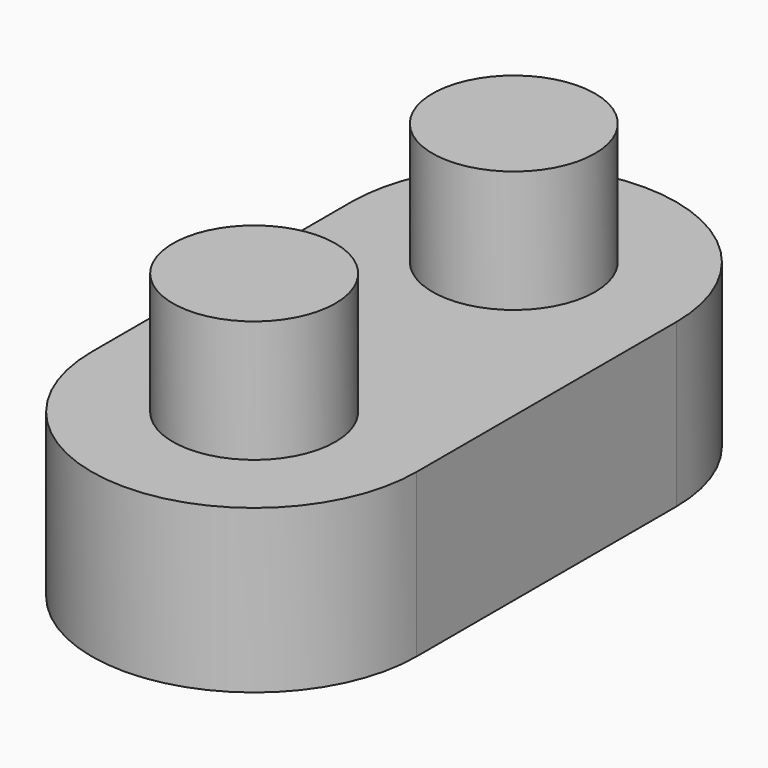
from build123d import *

# Parameters (mm, degrees)
F0_R     = 1
F1_DEPTH = 3.5
F2_DEPTH = 2
F3_DEPTH = 2


# Not quite as in the source:
# - a feature names something its author has since deleted; it is built from what else it names


with BuildPart() as f1:
    # F0 (on Top) → F1 (new body)
    with BuildSketch(Plane.XY):
        with Locations((-2.3999998812, 1.8953582125)):
            Circle(F0_R)
    extrude(amount=F1_DEPTH)



with BuildPart() as f1b:
    # F0 (on Top) → F1, piece 2 (new body)
    with BuildSketch(Plane.XY):
        with Locations((-2.3991598333, -2.1004185153)):
            Circle(F0_R)
    extrude(amount=F1_DEPTH)


with BuildPart() as f1_1:
    add(f1.part)

    add(f1b.part)  # F2 merges F1b
    # F0 (on Top) → F2 (join)
    with BuildSketch(Plane.XY):
        with BuildLine():
            ThreePointArc((-2.4958517574, -0.1027572147), (-3.8471556634, -0.7208141967), (-4.3991598333, -2.1004185153))
            ThreePointArc((-4.3991598333, -2.1004185153), (-2.3991598333, -4.1004185153), (-0.3991598333, -2.1004185153))
            ThreePointArc((-0.3991598333, -2.1004185153), (-0.9511640032, -0.7208141967), (-2.3024679093, -0.1027572147))
            ThreePointArc((-2.3024679093, -0.1027572147), (-2.3991598333, -0.1050959142), (-2.4958517574, -0.1027572147))
        make_face()
        with Locations((-2.3991598333, -2.1004185153)):
            Circle(F0_R, mode=Mode.SUBTRACT)
        with BuildLine():
            ThreePointArc((-2.3024679093, -0.1027572147), (-0.9511640032, -0.7208141967), (-0.3991598333, -2.1004185153))
            Line((-0.3991598333, -2.1004185153), (-0.3991598333, 1.8949040858))
            ThreePointArc((-0.3991598333, 1.8949040858), (-0.9511640032, 0.5152997672), (-2.3024679093, -0.1027572147))
        make_face()
        with BuildLine():
            ThreePointArc((-4.3991598333, 1.8949040858), (-3.8471556634, 0.5152997672), (-2.4958517574, -0.1027572147))
            ThreePointArc((-2.4958517574, -0.1027572147), (-2.3991598333, -0.1004185153), (-2.3024679093, -0.1027572147))
            ThreePointArc((-2.3024679093, -0.1027572147), (-0.9511640032, 0.5152997672), (-0.3991598333, 1.8949040858))
            ThreePointArc((-0.3991598333, 1.8949040858), (-2.3991598333, 3.8949040858), (-4.3991598333, 1.8949040858))
        make_face()
        with Locations((-2.3999998812, 1.8953582125)):
            Circle(F0_R, mode=Mode.SUBTRACT)
        with BuildLine():
            ThreePointArc((-2.3024679093, -0.1027572147), (-2.3991598333, -0.1004185153), (-2.4958517574, -0.1027572147))
            ThreePointArc((-2.4958517574, -0.1027572147), (-2.3991598333, -0.1050959142), (-2.3024679093, -0.1027572147))
        make_face()
    extrude(amount=F2_DEPTH)

    # F0 (on Top) → F3 (join)
    with BuildSketch(Plane.XY):
        with BuildLine():
            Line((-4.3991598333, 1.8949040858), (-4.3991598333, -2.1004185153))
            ThreePointArc((-4.3991598333, -2.1004185153), (-3.8471556634, -0.7208141967), (-2.4958517574, -0.1027572147))
            ThreePointArc((-2.4958517574, -0.1027572147), (-3.8471556634, 0.5152997672), (-4.3991598333, 1.8949040858))
        make_face()
    extrude(amount=F3_DEPTH)


solid = f1_1.part
